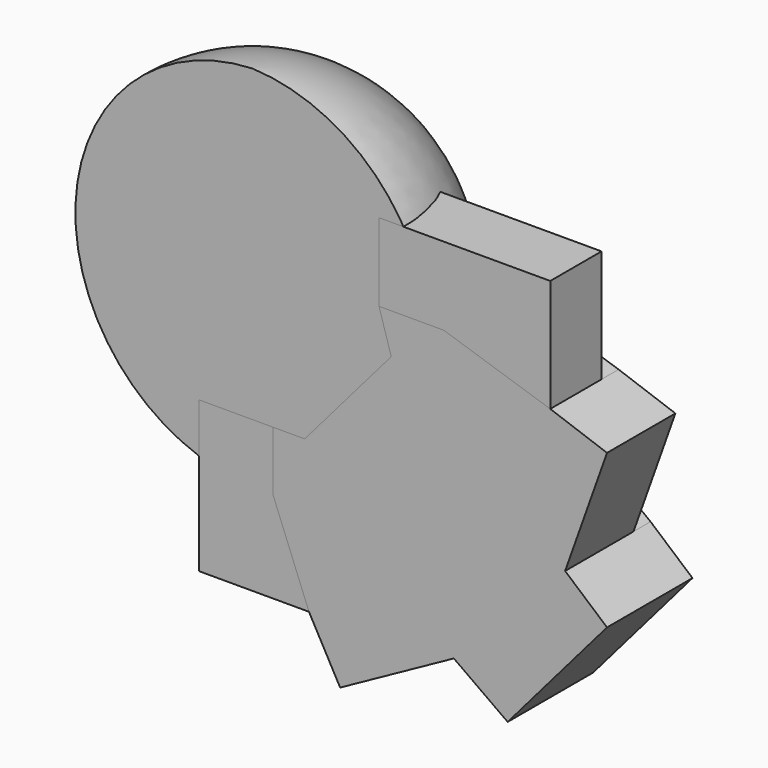
from build123d import *

# Parameters (mm, degrees)
F1_ANGLE = 180
F2_DEPTH = 12.7
F3_DEPTH = 10.16
F4_DEPTH = 7.62


with BuildPart() as f1:
    # F0 (on Front) → F1 (revolve)
    with BuildSketch(Plane.XZ):
        with BuildLine():
            ThreePointArc((-5.2119125612, 24.1178274155), (-26.0229998372, 5.420144988), (-11.5379225463, -18.5149175279))
            Line((-11.5379225463, -18.5149175279), (-11.5379225463, -12.6310279712))
            Line((-11.5379225463, -12.6310279712), (-5.2119125612, -12.6310279712))
            Line((-5.2119125612, -12.6310279712), (-5.2119125612, 24.1178274155))
        make_face()
        with BuildLine():
            Line((-11.5379225463, -12.6310279712), (-11.5379225463, -18.5149175279))
            ThreePointArc((-11.5379225463, -18.5149175279), (-8.4192556337, -19.3491942107), (-5.2119125612, -19.7166874899))
            Line((-5.2119125612, -19.7166874899), (-5.2119125612, -12.6310279712))
            Line((-5.2119125612, -12.6310279712), (-11.5379225463, -12.6310279712))
        make_face()
    revolve(axis=Axis((-5.2119125612, 0, 2.2005699628), (0, 0, -1)), revolution_arc=F1_ANGLE)


with BuildPart() as f2:
    # F0 (on Front) → F2 (new body)
    with BuildSketch(Plane.XZ):
        with BuildLine():
            Line((5.6357962208, -17.3423814325), (18.7385064086, -29.8429892095))
            Line((18.7385064086, -29.8429892095), (25.1361876726, -34.4077348709))
            Line((25.1361876726, -34.4077348709), (36.948826164, -20.6721108407))
            Line((36.948826164, -20.6721108407), (31.9681242528, -16.3887065352))
            Line((31.9681242528, -16.3887065352), (16.5153805091, -4.6415458401))
            ThreePointArc((16.5153805091, -4.6415458401), (12.3334800243, -12.0694784371), (5.6357962208, -17.3423814325))
        make_face()
        with BuildLine():
            Line((1.0108276248, -12.6310279712), (5.6357962208, -17.3423814325))
            ThreePointArc((5.6357962208, -17.3423814325), (12.3334800243, -12.0694784371), (16.5153805091, -4.6415458401))
            Line((16.5153805091, -4.6415458401), (11.2948295207, -0.6728880797))
            Line((11.2948295207, -0.6728880797), (1.0108276248, -12.6310279712))
        make_face()
    extrude(amount=-F2_DEPTH)

    # F0 (on Front) → F3 (join)
    with BuildSketch(Plane.XZ):
        with BuildLine():
            ThreePointArc((17.6097934393, 2.2005699628), (17.5887807067, 3.1604629732), (17.525782767, 4.1185169309))
            Line((17.525782767, 4.1185169309), (9.8418733105, 4.1185169309))
            Line((9.8418733105, 4.1185169309), (11.2948295207, -0.6728880797))
            Line((11.2948295207, -0.6728880797), (16.5153805091, -4.6415458401))
            ThreePointArc((16.5153805091, -4.6415458401), (17.3344622227, -1.2639750406), (17.6097934393, 2.2005699628))
        make_face()
        with BuildLine():
            Line((-2.7701762575, -12.6310279712), (-2.7701762575, -19.679407769))
            ThreePointArc((-2.7701762575, -19.679407769), (1.5501772882, -18.933049171), (5.6357962208, -17.3423814325))
            Line((5.6357962208, -17.3423814325), (1.0108276248, -12.6310279712))
            Line((1.0108276248, -12.6310279712), (-2.7701762575, -12.6310279712))
        make_face()
        with BuildLine():
            Line((-2.7701762575, -19.679407769), (1.5109189553, -30.5617600679))
            Line((1.5109189553, -30.5617600679), (5.2195368335, -37.2922159731))
            Line((5.2195368335, -37.2922159731), (18.7385064086, -29.8429892095))
            Line((18.7385064086, -29.8429892095), (5.6357962208, -17.3423814325))
            ThreePointArc((5.6357962208, -17.3423814325), (1.5501772882, -18.933049171), (-2.7701762575, -19.679407769))
        make_face()
        with BuildLine():
            Line((30.1995456827, 0), (17.525782767, 4.1185169309))
            ThreePointArc((17.525782767, 4.1185169309), (17.5887807067, 3.1604629732), (17.6097934393, 2.2005699628))
            ThreePointArc((17.6097934393, 2.2005699628), (17.3344622227, -1.2639750406), (16.5153805091, -4.6415458401))
            Line((16.5153805091, -4.6415458401), (31.9681242528, -16.3887065352))
            Line((31.9681242528, -16.3887065352), (36.948826164, -2.403734019))
            Line((36.948826164, -2.403734019), (30.1995456827, 0))
        make_face()
    extrude(amount=-F3_DEPTH)


with BuildPart() as f4:
    # F0 (on Front) → F4 (new body)
    with BuildSketch(Plane.XZ):
        with BuildLine():
            ThreePointArc((17.525782767, 4.1185169309), (16.5542154561, 8.9232435656), (14.5398945858, 13.3922314271))
            Line((14.5398945858, 13.3922314271), (9.8418733105, 13.3922314271))
            Line((9.8418733105, 13.3922314271), (9.8418733105, 4.1185169309))
            Line((9.8418733105, 4.1185169309), (17.525782767, 4.1185169309))
        make_face()
        with BuildLine():
            Line((16.2080340087, 13.3922314271), (14.5398945858, 13.3922314271))
            ThreePointArc((14.5398945858, 13.3922314271), (16.5542154561, 8.9232435656), (17.525782767, 4.1185169309))
            Line((17.525782767, 4.1185169309), (30.1995456827, 0))
            Line((30.1995456827, 0), (30.1995456827, 13.3922314271))
            Line((30.1995456827, 13.3922314271), (16.2080340087, 13.3922314271))
        make_face()
    extrude(amount=-F4_DEPTH)


with BuildPart() as f4b:
    # F0 (on Front) → F4, piece 2 (new body)
    with BuildSketch(Plane.XZ):
        with BuildLine():
            Line((-11.5379225463, -18.5149175279), (-11.5379225463, -19.2985497415))
            Line((-11.5379225463, -19.2985497415), (-11.5379225463, -30.5617600679))
            Line((-11.5379225463, -30.5617600679), (1.5109189553, -30.5617600679))
            Line((1.5109189553, -30.5617600679), (-2.7701762575, -19.679407769))
            ThreePointArc((-2.7701762575, -19.679407769), (-3.9905252177, -19.7320534894), (-5.2119125612, -19.7166874899))
            ThreePointArc((-5.2119125612, -19.7166874899), (-8.4192556337, -19.3491942107), (-11.5379225463, -18.5149175279))
        make_face()
        with BuildLine():
            Line((-11.5379225463, -12.6310279712), (-11.5379225463, -18.5149175279))
            ThreePointArc((-11.5379225463, -18.5149175279), (-8.4192556337, -19.3491942107), (-5.2119125612, -19.7166874899))
            Line((-5.2119125612, -19.7166874899), (-5.2119125612, -12.6310279712))
            Line((-5.2119125612, -12.6310279712), (-11.5379225463, -12.6310279712))
        make_face()
        with BuildLine():
            Line((-5.2119125612, -12.6310279712), (-5.2119125612, -19.7166874899))
            ThreePointArc((-5.2119125612, -19.7166874899), (-3.9905252177, -19.7320534894), (-2.7701762575, -19.679407769))
            Line((-2.7701762575, -19.679407769), (-2.7701762575, -12.6310279712))
            Line((-2.7701762575, -12.6310279712), (-5.2119125612, -12.6310279712))
        make_face()
    extrude(amount=-F4_DEPTH)


solid = Compound([f1.part, f2.part, f4.part, f4b.part])
